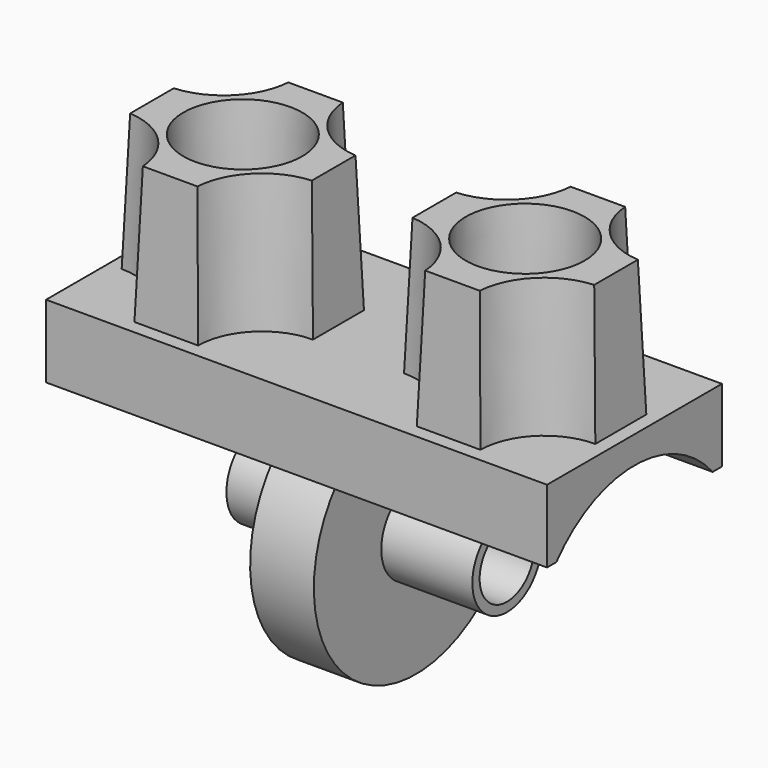
from build123d import *

# Parameters (mm, degrees)
F0_W                    = 55
F0_H                    = 24
F1_DEPTH                = 8
F3_DEPTH                = 60
F4_R                    = 14
F5_DEPTH                = 3.5
F5_DEPTH_BACK           = 3.5
F6_R                    = 4.75
F6_R_2                  = 3.75
F7_DEPTH                = 10
F9_R                    = 6
F10_DEPTH               = 15
DRAFT_F10_DRAFTED_ANGLE = 2


# Not quite as in the source:
# - an extrude with a draft is written as a straight extrude whose walls are then drafted


with BuildPart() as f1:
    # F0 (on Top) → F1 (new body)
    with BuildSketch(Plane.XY):
        Rectangle(F0_W, F0_H)
    extrude(amount=F1_DEPTH)

    # F2 (on face) → F3 (cut)
    with BuildSketch(Plane.YZ.offset(27.5)):
        with BuildLine():
            Line((-10.7238052948, 0), (10.7238052948, 0))
            ThreePointArc((10.7238052948, 0), (0, 5), (-10.7238052948, 0))
        make_face()
    extrude(amount=-F3_DEPTH, mode=Mode.SUBTRACT)

    # F4 (on Right) → F5 (join, two sides)
    with BuildSketch(Plane.YZ) as f5_sk:
        with Locations((0, -9)):
            Circle(F4_R)
    extrude(amount=F5_DEPTH)
    extrude(f5_sk.sketch, amount=-F5_DEPTH_BACK)

    # F6 (on face) → F7 (join)
    with BuildSketch(Plane.YZ.offset(3.5)):
        with Locations((0, -9)):
            Circle(F6_R)
        with Locations((0, -9)):
            Circle(F6_R_2, mode=Mode.SUBTRACT)
    extrude(amount=F7_DEPTH)

    # F8: F1 across plane


with BuildPart() as f1_1:
    add(f1.part)
    add(f1.part.mirror(Plane.YZ))


with BuildPart() as f10_drafted:
    # F9 (on face) → F10 (new body)
    with BuildSketch(Plane.XY.offset(8)):
        with BuildLine():
            Line((19, 10.5), (12, 10.5))
            ThreePointArc((12, 10.5), (9.9497474683, 5.5502525317), (5, 3.5))
            Line((5, 3.5), (5, -3.5))
            ThreePointArc((5, -3.5), (9.9497474683, -5.5502525317), (12, -10.5))
            Line((12, -10.5), (19, -10.5))
            ThreePointArc((19, -10.5), (21.0502525317, -5.5502525317), (26, -3.5))
            Line((26, -3.5), (26, 3.5))
            ThreePointArc((26, 3.5), (21.0502525317, 5.5502525317), (19, 10.5))
        make_face()
        with Locations((15.5, 0)):
            Circle(F9_R, mode=Mode.SUBTRACT)
    extrude(amount=F10_DEPTH)

    # draft_F10_drafted
    draft_f10_drafted_walls = [f10_drafted.faces().sort_by_distance(p)[0] for p in [
        (21.0502525317, 5.5502525317, 18),
        (15.5, 10.5, 18),
        (9.9497474683, 5.5502525317, 18),
        (5, 0, 18),
        (9.9497474683, -5.5502525317, 18),
        (15.5, -10.5, 18),
        (21.0502525317, -5.5502525317, 18),
        (26, 0, 18),
        (9.5, 0, 18),
    ]]
    draft(draft_f10_drafted_walls, neutral_plane=Plane.XY.offset(8), angle=DRAFT_F10_DRAFTED_ANGLE)


with BuildPart() as f1_2:
    add(f1_1.part)

    # join_F10_drafted: union F10_drafted
    add(f10_drafted.part)

    # F11: F1 across plane


with BuildPart() as f1_3:
    add(f1_2.part)
    add(f1_2.part.mirror(Plane.YZ))


solid = f1_3.part
